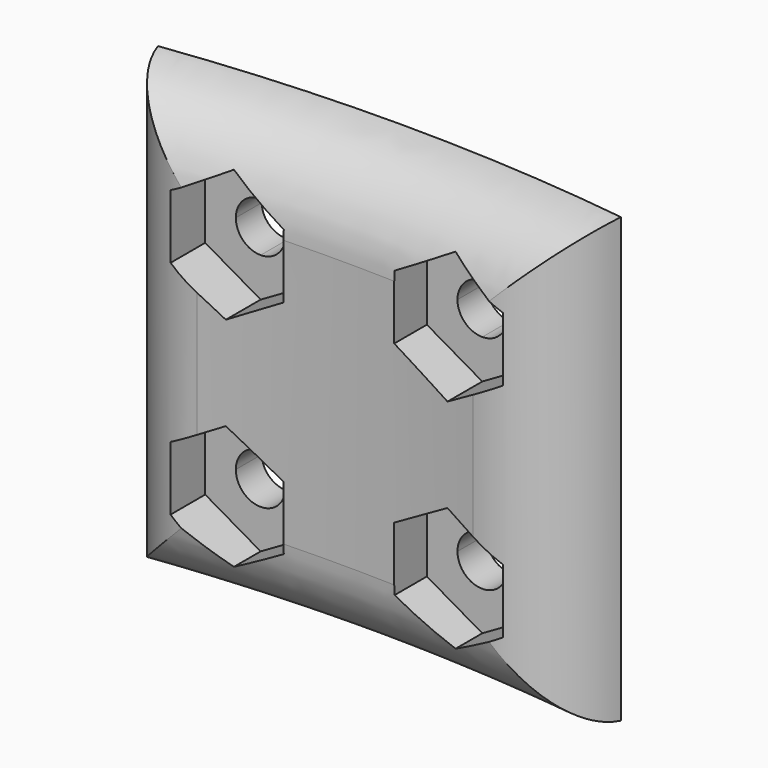
from build123d import *

# Parameters (mm, degrees)
F1_DEPTH    = 12.7
F6_DEPTH    = 25.4
F7_T1_DEPTH = 49.4232912098
F7_T4_ANGLE = 29.8619681209
F7_T6_ANGLE = 29.8619681209
F8_START    = -2.159
F8_DEPTH    = 23.241
F9_DEPTH    = 25.4


# Not quite as in the source:
# - a fillet or chamfer that OpenCascade refuses, or shapes differently, is made with other operations: its cross-section is extruded or revolved along the edge and cut away or added


with BuildPart() as f1:
    # F0 (on Top) → F1 (new body, symmetric)
    with BuildSketch(Plane.XY):
        with BuildLine():
            ThreePointArc((0, 101.6), (-6.6449579298, 101.382466601), (-13.2614611296, 100.7307979156))
            Line((-13.2614611296, 100.7307979156), (-12.6812722051, 96.3238255068))
            ThreePointArc((-12.6812722051, 96.3238255068), (-6.3542410204, 96.9469836872), (0, 97.155))
            Line((0, 97.155), (0, 101.6))
        make_face()
        with BuildLine():
            Line((12.6812722051, 96.3238255068), (13.2614611296, 100.7307979156))
            ThreePointArc((13.2614611296, 100.7307979156), (6.6449579298, 101.382466601), (0, 101.6))
            Line((0, 101.6), (0, 97.155))
            ThreePointArc((0, 97.155), (6.3542410204, 96.9469836872), (12.6812722051, 96.3238255068))
        make_face()
    extrude(amount=F1_DEPTH, both=True)

    # F5 (on line) → F6 (cut)
    with BuildSketch(Plane(origin=(0, 101.6, 0), x_dir=(-1, 0, 0), z_dir=(0, 1, 0))):
        with BuildLine():
            Line((6.35, -6.35), (4.9276, -6.35))
            ThreePointArc((4.9276, -6.35), (6.35, -7.7724), (7.7724, -6.35))
            ThreePointArc((7.7724, -6.35), (7.3557886856, -5.3442113144), (6.35, -4.9276))
            Line((6.35, -4.9276), (6.35, -6.35))
        make_face()
        with BuildLine():
            ThreePointArc((6.35, -4.9276), (5.3442113144, -5.3442113144), (4.9276, -6.35))
            Line((4.9276, -6.35), (6.35, -6.35))
            Line((6.35, -6.35), (6.35, -4.9276))
        make_face()
        with BuildLine():
            Line((-4.9276, -6.35), (-6.35, -6.35))
            Line((-6.35, -6.35), (-6.35, -4.9276))
            ThreePointArc((-6.35, -4.9276), (-7.3557886856, -7.3557886856), (-4.9276, -6.35))
        make_face()
        with BuildLine():
            Line((-6.35, -4.9276), (-6.35, -6.35))
            Line((-6.35, -6.35), (-4.9276, -6.35))
            ThreePointArc((-4.9276, -6.35), (-5.3442113144, -5.3442113144), (-6.35, -4.9276))
        make_face()
        with BuildLine():
            Line((6.35, 6.35), (6.35, 4.9276))
            ThreePointArc((6.35, 4.9276), (7.3557886856, 5.3442113144), (7.7724, 6.35))
            ThreePointArc((7.7724, 6.35), (6.35, 7.7724), (4.9276, 6.35))
            Line((4.9276, 6.35), (6.35, 6.35))
        make_face()
        with BuildLine():
            ThreePointArc((4.9276, 6.35), (5.3442113144, 5.3442113144), (6.35, 4.9276))
            Line((6.35, 4.9276), (6.35, 6.35))
            Line((6.35, 6.35), (4.9276, 6.35))
        make_face()
        with BuildLine():
            ThreePointArc((-4.9276, 6.35), (-7.3557886856, 7.3557886856), (-6.35, 4.9276))
            Line((-6.35, 4.9276), (-6.35, 6.35))
            Line((-6.35, 6.35), (-4.9276, 6.35))
        make_face()
        with BuildLine():
            Line((-6.35, 6.35), (-6.35, 4.9276))
            ThreePointArc((-6.35, 4.9276), (-5.3442113144, 5.3442113144), (-4.9276, 6.35))
            Line((-4.9276, 6.35), (-6.35, 6.35))
        make_face()
    extrude(amount=-F6_DEPTH, mode=Mode.SUBTRACT)

    # F7: fillet of radius 5.08 on 4 edges, made by hand

    # F7_s2 → F7_t1 (cut)
    with BuildSketch(Plane.XY.offset(-24.7116456049)):
        with BuildLine():
            ThreePointArc((7.9036679621, 96.8329802172), (11.3054660928, 97.7882158705), (13.2614611296, 100.7307979156))
            Line((13.2614611296, 100.7307979156), (12.6812722051, 96.3238255068))
            ThreePointArc((12.6812722051, 96.3238255068), (10.2956180024, 96.6079410553), (7.9036679621, 96.8329802172))
        make_face()
        with BuildLine():
            ThreePointArc((-7.9036679621, 96.8329802172), (-11.3054660928, 97.7882158705), (-13.2614611296, 100.7307979156))
            Line((-13.2614611296, 100.7307979156), (-12.6812722051, 96.3238255068))
            ThreePointArc((-12.6812722051, 96.3238255068), (-10.2956180024, 96.6079410553), (-7.9036679621, 96.8329802172))
        make_face()
    extrude(amount=F7_T1_DEPTH, mode=Mode.SUBTRACT)

    # F7_s3 → F7_t4 (revolve, cut)
    with BuildSketch(Plane(origin=(0, 0, 0), x_dir=(0, 0, 1), z_dir=(-0.9662368873, -0.2576553465, 0))):
        with BuildLine():
            ThreePointArc((7.6598437524, 97.155), (11.0199479175, 98.425), (12.7, 101.6))
            Line((12.7, 101.6), (12.7, 97.155))
            Line((12.7, 97.155), (7.6598437524, 97.155))
        make_face()
    revolve(axis=Axis((0, 0, 12.7), (0, 0, -1)), revolution_arc=F7_T4_ANGLE, mode=Mode.SUBTRACT)

    # F7_s5 → F7_t6 (revolve, cut)
    with BuildSketch(Plane(origin=(0, 0, 0), x_dir=(0, 0, 1), z_dir=(-0.9662368873, -0.2576553465, 0))):
        with BuildLine():
            ThreePointArc((-7.6598437524, 97.155), (-11.0199479175, 98.425), (-12.7, 101.6))
            Line((-12.7, 101.6), (-12.7, 97.155))
            Line((-12.7, 97.155), (-7.6598437524, 97.155))
        make_face()
    revolve(axis=Axis((0, 0, -12.7), (0, 0, -1)), revolution_arc=F7_T6_ANGLE, mode=Mode.SUBTRACT)

    # F5 (on line) → F8 (cut)
    with BuildSketch(Plane(origin=(0, 101.6, 0), x_dir=(-1, 0, 0), z_dir=(0, 1, 0)).offset(F8_START)):
        with BuildLine():
            Line((6.35, 4.9276), (6.35, 2.6838257906))
            Line((6.35, 2.6838257906), (9.525, 4.5169128953))
            Line((9.525, 4.5169128953), (9.525, 8.1830871047))
            Line((9.525, 8.1830871047), (6.35, 10.0161742094))
            Line((6.35, 10.0161742094), (3.175, 8.1830871047))
            Line((3.175, 8.1830871047), (3.175, 6.35))
            Line((3.175, 6.35), (4.9276, 6.35))
            ThreePointArc((4.9276, 6.35), (6.35, 7.7724), (7.7724, 6.35))
            ThreePointArc((7.7724, 6.35), (7.3557886856, 5.3442113144), (6.35, 4.9276))
        make_face()
        with BuildLine():
            Line((3.175, 4.5169128953), (6.35, 2.6838257906))
            Line((6.35, 2.6838257906), (6.35, 4.9276))
            ThreePointArc((6.35, 4.9276), (5.3442113144, 5.3442113144), (4.9276, 6.35))
            Line((4.9276, 6.35), (3.175, 6.35))
            Line((3.175, 6.35), (3.175, 4.5169128953))
        make_face()
        with BuildLine():
            Line((4.9276, -6.35), (3.175, -6.35))
            Line((3.175, -6.35), (3.175, -8.1830871047))
            Line((3.175, -8.1830871047), (6.35, -10.0161742094))
            Line((6.35, -10.0161742094), (9.525, -8.1830871047))
            Line((9.525, -8.1830871047), (9.525, -4.5169128953))
            Line((9.525, -4.5169128953), (6.35, -2.6838257906))
            Line((6.35, -2.6838257906), (6.35, -4.9276))
            ThreePointArc((6.35, -4.9276), (7.3557886856, -5.3442113144), (7.7724, -6.35))
            ThreePointArc((7.7724, -6.35), (6.35, -7.7724), (4.9276, -6.35))
        make_face()
        with BuildLine():
            Line((3.175, -4.5169128953), (3.175, -6.35))
            Line((3.175, -6.35), (4.9276, -6.35))
            ThreePointArc((4.9276, -6.35), (5.3442113144, -5.3442113144), (6.35, -4.9276))
            Line((6.35, -4.9276), (6.35, -2.6838257906))
            Line((6.35, -2.6838257906), (3.175, -4.5169128953))
        make_face()
        with BuildLine():
            Line((-3.175, -6.35), (-4.9276, -6.35))
            ThreePointArc((-4.9276, -6.35), (-7.3557886856, -7.3557886856), (-6.35, -4.9276))
            Line((-6.35, -4.9276), (-6.35, -2.6838257906))
            Line((-6.35, -2.6838257906), (-9.525, -4.5169128953))
            Line((-9.525, -4.5169128953), (-9.525, -8.1830871047))
            Line((-9.525, -8.1830871047), (-6.35, -10.0161742094))
            Line((-6.35, -10.0161742094), (-3.175, -8.1830871047))
            Line((-3.175, -8.1830871047), (-3.175, -6.35))
        make_face()
        with BuildLine():
            ThreePointArc((-6.35, -4.9276), (-5.3442113144, -5.3442113144), (-4.9276, -6.35))
            Line((-4.9276, -6.35), (-3.175, -6.35))
            Line((-3.175, -6.35), (-3.175, -4.5169128953))
            Line((-3.175, -4.5169128953), (-6.35, -2.6838257906))
            Line((-6.35, -2.6838257906), (-6.35, -4.9276))
        make_face()
        with BuildLine():
            Line((-6.35, 4.9276), (-6.35, 2.6838257906))
            Line((-6.35, 2.6838257906), (-3.175, 4.5169128953))
            Line((-3.175, 4.5169128953), (-3.175, 6.35))
            Line((-3.175, 6.35), (-4.9276, 6.35))
            ThreePointArc((-4.9276, 6.35), (-5.3442113144, 5.3442113144), (-6.35, 4.9276))
        make_face()
        with BuildLine():
            Line((-9.525, 4.5169128953), (-6.35, 2.6838257906))
            Line((-6.35, 2.6838257906), (-6.35, 4.9276))
            ThreePointArc((-6.35, 4.9276), (-7.3557886856, 7.3557886856), (-4.9276, 6.35))
            Line((-4.9276, 6.35), (-3.175, 6.35))
            Line((-3.175, 6.35), (-3.175, 8.1830871047))
            Line((-3.175, 8.1830871047), (-6.35, 10.0161742094))
            Line((-6.35, 10.0161742094), (-9.525, 8.1830871047))
            Line((-9.525, 8.1830871047), (-9.525, 4.5169128953))
        make_face()
    extrude(amount=-F8_DEPTH, mode=Mode.SUBTRACT)

    # F5 (on line) → F9 (cut)
    with BuildSketch(Plane(origin=(0, 101.6, 0), x_dir=(-1, 0, 0), z_dir=(0, 1, 0))):
        with BuildLine():
            ThreePointArc((-4.9276, 6.35), (-7.3557886856, 7.3557886856), (-6.35, 4.9276))
            Line((-6.35, 4.9276), (-6.35, 6.35))
            Line((-6.35, 6.35), (-4.9276, 6.35))
        make_face()
        with BuildLine():
            Line((-6.35, 6.35), (-6.35, 4.9276))
            ThreePointArc((-6.35, 4.9276), (-5.3442113144, 5.3442113144), (-4.9276, 6.35))
            Line((-4.9276, 6.35), (-6.35, 6.35))
        make_face()
    extrude(amount=-F9_DEPTH, mode=Mode.SUBTRACT)


solid = f1.part
